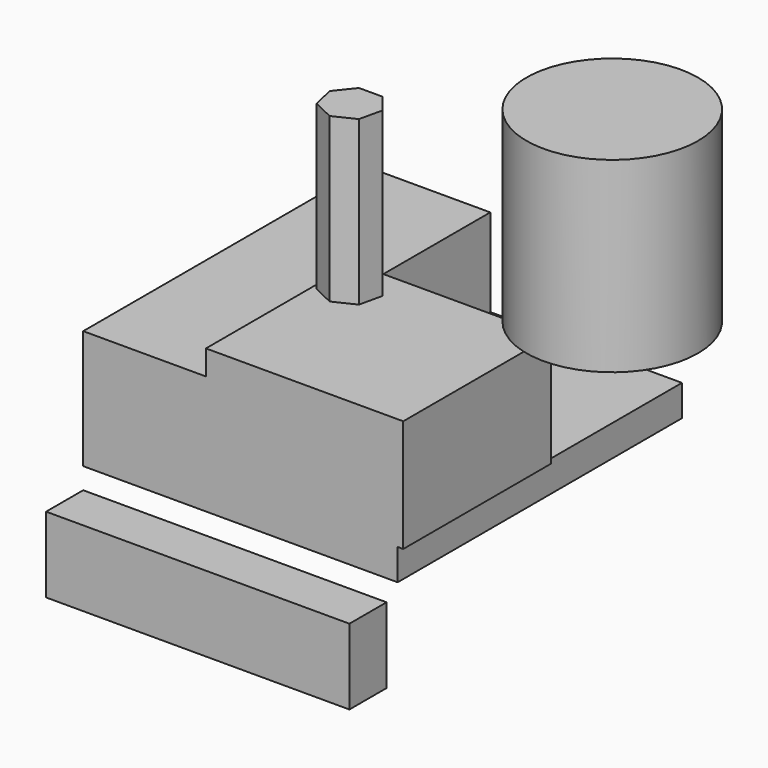
from build123d import *

# Parameters (mm, degrees)
F0_R      = 46.9601079777
F1_DEPTH  = 102.362
F2_W      = 108.0089695752
F2_H      = 61.5570303053
F3_DEPTH  = 101.092
F5_DEPTH  = 89.408
F10_DEPTH = 194.564
F11_W     = 166.0638004541
F11_H     = 41.3593128324
F12_DEPTH = 25.4


# Not quite as in the source:
# - the program builds the solid bodies; features that only make, move or delete a surface that nothing else refers to are left out


with BuildPart() as f1:
    # F0 (on Top) → F1 (new body)
    with BuildSketch(Plane.XY):
        with Locations((-7.1760101607, -2.244985865)):
            Circle(F0_R)
    extrude(amount=F1_DEPTH)


with BuildPart() as f3:
    # F2 (on Front) → F3 (new body)
    with BuildSketch(Plane.XZ):
        with Locations((-96.5330209583, -50.1435371116)):
            Rectangle(F2_W, F2_H)
    extrude(amount=F3_DEPTH)

    # F9 (on face) → F10 (join)
    with BuildSketch(Plane.XZ.offset(101.092)):
        Polygon((-150.5375057459, -32.8971557319), (-217.7324593067, -32.8971557319), (-217.7324593067, -97.96436131), (-45.5931425095, -97.96436131), (-45.5931425095, -80.9220522642), (-150.5375057459, -80.9220522642), align=None)
    extrude(amount=-F10_DEPTH)


with BuildPart() as f5:
    # F4 (on Top) → F5 (new body)
    with BuildSketch(Plane.XY):
        Polygon((-106.7080545129, -35.1148024201), (-119.5374381838, -35.1148024201), (-127.5364280668, -45.1452184747), (-124.6816216302, -57.6529427116), (-113.1227463484, -63.2194036693), (-101.5638710665, -57.6529427116), (-98.70906463, -45.1452184747), align=None)
    extrude(amount=F5_DEPTH)


with BuildPart() as f12:
    # F11 (on face) → F12 (new body)
    with BuildSketch(Plane.XZ.offset(101.092)):
        with Locations((-134.7005590796, -130.2479021251)):
            Rectangle(F11_W, F11_H)
    extrude(amount=F12_DEPTH)


solid = Compound([f1.part, f3.part, f5.part, f12.part])
